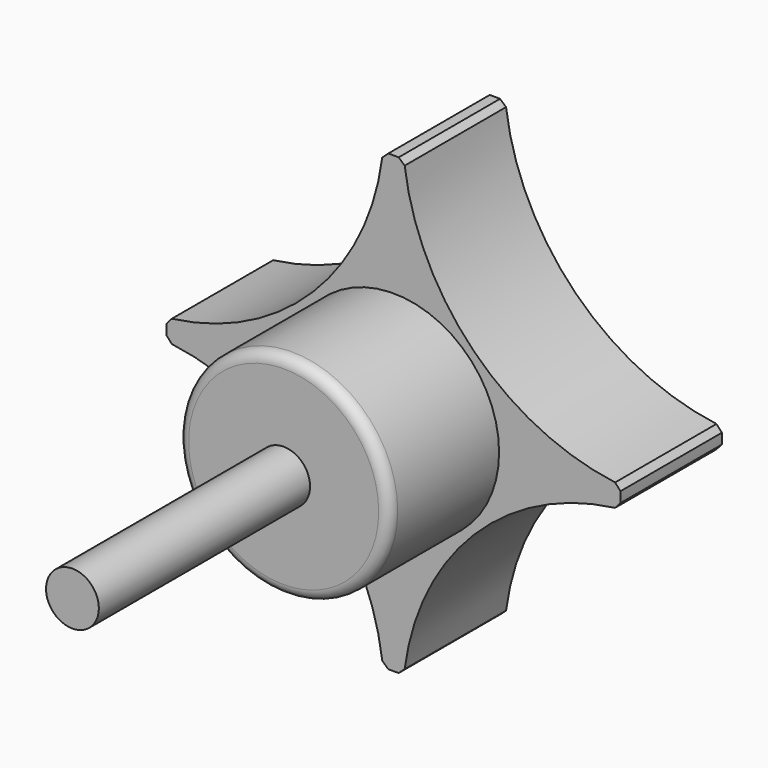
from build123d import *

# Parameters (mm, degrees)
F0_R        = 21.5
F1_DEPTH    = 12
F3_DEPTH    = 12
F4_R        = 10
F5_DEPTH    = 13
F6_R        = 2.5
F7_DEPTH    = 25
F8_T1_DEPTH = 14.6145321273
F9_R        = 1


# Not quite as in the source:
# - a fillet or chamfer that OpenCascade refuses, or shapes differently, is made with other operations: its cross-section is extruded or revolved along the edge and cut away or added


with BuildPart() as f1:
    # F0 (on Front) → F1 (new body)
    with BuildSketch(Plane.XZ):
        Circle(F0_R)
    extrude(amount=F1_DEPTH)

    # F2 (on face) → F3 (cut)
    with BuildSketch(Plane.XZ.offset(12)):
        with BuildLine():
            ThreePointArc((-1, 21.4767315949), (-15.2027957955, 15.2027957955), (-21.4767315949, 1))
            ThreePointArc((-21.4767315949, 1), (-7.6309801067, 7.6309801067), (-1, 21.4767315949))
        make_face()
        with BuildLine():
            ThreePointArc((1, 21.4767315949), (7.6309801067, 7.6309801067), (21.4767315949, 1))
            ThreePointArc((21.4767315949, 1), (15.2027957955, 15.2027957955), (1, 21.4767315949))
        make_face()
        with BuildLine():
            ThreePointArc((-1, -21.4767315949), (-7.6309801067, -7.6309801067), (-21.4767315949, -1))
            ThreePointArc((-21.4767315949, -1), (-15.2027957955, -15.2027957955), (-1, -21.4767315949))
        make_face()
        with BuildLine():
            ThreePointArc((1, -21.4767315949), (15.2027957955, -15.2027957955), (21.4767315949, -1))
            ThreePointArc((21.4767315949, -1), (7.6309801067, -7.6309801067), (1, -21.4767315949))
        make_face()
    extrude(amount=-F3_DEPTH, mode=Mode.SUBTRACT)

    # F4 (on face) → F5 (join)
    with BuildSketch(Plane.XZ.offset(12)):
        Circle(F4_R)
    extrude(amount=F5_DEPTH)

    # F6 (on face) → F7 (join)
    with BuildSketch(Plane.XZ.offset(25)):
        Circle(F6_R)
    extrude(amount=F7_DEPTH)

    # F8: chamfer of 0.5 on 8 edges, made by hand

    # F8_s2 → F8_t1 (cut)
    with BuildSketch(Plane.XZ.offset(-1.3072660637)):
        with BuildLine():
            Line((-0.4780125983, 21.5077200164), (-1.0733486412, 20.9725576393))
            Line((-1.0733486412, 20.9725576393), (-1.0832651887, 20.973846858))
            ThreePointArc((-1.0832651887, 20.973846858), (-1.0387448634, 21.2248919874), (-1.0099418634, 21.4778083267))
            Line((-1.0099418634, 21.4778083267), (-1.0004651163, 21.4867207724))
            ThreePointArc((-1.0004651163, 21.4867207724), (-0.7391806182, 21.4972954581), (-0.4782418478, 21.5177173883))
            Line((-0.4782418478, 21.5177173883), (-0.4780125983, 21.5077200164))
        make_face()
        with BuildLine():
            Line((-20.9725576393, 1.0733486412), (-21.5077200164, 0.4780125983))
            Line((-21.5077200164, 0.4780125983), (-21.5177173883, 0.4782418478))
            ThreePointArc((-21.5177173883, 0.4782418478), (-21.4972954581, 0.7391806182), (-21.4867207724, 1.0004651163))
            Line((-21.4867207724, 1.0004651163), (-21.4778083267, 1.0099418634))
            ThreePointArc((-21.4778083267, 1.0099418634), (-21.2248919874, 1.0387448634), (-20.973846858, 1.0832651887))
            Line((-20.973846858, 1.0832651887), (-20.9725576393, 1.0733486412))
        make_face()
        with BuildLine():
            Line((-21.5077200164, -0.4780125983), (-20.9725576393, -1.0733486412))
            Line((-20.9725576393, -1.0733486412), (-20.973846858, -1.0832651887))
            ThreePointArc((-20.973846858, -1.0832651887), (-21.2248919874, -1.0387448634), (-21.4778083267, -1.0099418634))
            Line((-21.4778083267, -1.0099418634), (-21.4867207724, -1.0004651163))
            ThreePointArc((-21.4867207724, -1.0004651163), (-21.4972954581, -0.7391806182), (-21.5177173883, -0.4782418478))
            Line((-21.5177173883, -0.4782418478), (-21.5077200164, -0.4780125983))
        make_face()
        with BuildLine():
            Line((1.0733486412, 20.9725576393), (0.4780125983, 21.5077200164))
            Line((0.4780125983, 21.5077200164), (0.4782418478, 21.5177173883))
            ThreePointArc((0.4782418478, 21.5177173883), (0.7391806182, 21.4972954581), (1.0004651163, 21.4867207724))
            Line((1.0004651163, 21.4867207724), (1.0099418634, 21.4778083267))
            ThreePointArc((1.0099418634, 21.4778083267), (1.0387448634, 21.2248919874), (1.0832651887, 20.973846858))
            Line((1.0832651887, 20.973846858), (1.0733486412, 20.9725576393))
        make_face()
        with BuildLine():
            Line((21.5077200164, 0.4780125983), (20.9725576393, 1.0733486412))
            Line((20.9725576393, 1.0733486412), (20.973846858, 1.0832651887))
            ThreePointArc((20.973846858, 1.0832651887), (21.2248919874, 1.0387448634), (21.4778083267, 1.0099418634))
            Line((21.4778083267, 1.0099418634), (21.4867207724, 1.0004651163))
            ThreePointArc((21.4867207724, 1.0004651163), (21.4972954581, 0.7391806182), (21.5177173883, 0.4782418478))
            Line((21.5177173883, 0.4782418478), (21.5077200164, 0.4780125983))
        make_face()
        with BuildLine():
            Line((1.0733486412, -20.9725576393), (0.4780125983, -21.5077200164))
            Line((0.4780125983, -21.5077200164), (0.4782418478, -21.5177173883))
            ThreePointArc((0.4782418478, -21.5177173883), (0.7391806182, -21.4972954581), (1.0004651163, -21.4867207724))
            Line((1.0004651163, -21.4867207724), (1.0099418634, -21.4778083267))
            ThreePointArc((1.0099418634, -21.4778083267), (1.0387448634, -21.2248919874), (1.0832651887, -20.973846858))
            Line((1.0832651887, -20.973846858), (1.0733486412, -20.9725576393))
        make_face()
        with BuildLine():
            Line((-1.0733486412, -20.9725576393), (-0.4780125983, -21.5077200164))
            Line((-0.4780125983, -21.5077200164), (-0.4782418478, -21.5177173883))
            ThreePointArc((-0.4782418478, -21.5177173883), (-0.7391806182, -21.4972954581), (-1.0004651163, -21.4867207724))
            Line((-1.0004651163, -21.4867207724), (-1.0099418634, -21.4778083267))
            ThreePointArc((-1.0099418634, -21.4778083267), (-1.0387448634, -21.2248919874), (-1.0832651887, -20.973846858))
            Line((-1.0832651887, -20.973846858), (-1.0733486412, -20.9725576393))
        make_face()
        with BuildLine():
            Line((21.5077200164, -0.4780125983), (20.9725576393, -1.0733486412))
            Line((20.9725576393, -1.0733486412), (20.973846858, -1.0832651887))
            ThreePointArc((20.973846858, -1.0832651887), (21.2248919874, -1.0387448634), (21.4778083267, -1.0099418634))
            Line((21.4778083267, -1.0099418634), (21.4867207724, -1.0004651163))
            ThreePointArc((21.4867207724, -1.0004651163), (21.4972954581, -0.7391806182), (21.5177173883, -0.4782418478))
            Line((21.5177173883, -0.4782418478), (21.5077200164, -0.4780125983))
        make_face()
    extrude(amount=F8_T1_DEPTH, mode=Mode.SUBTRACT)

    # F9
    f9_edges = [f1.edges().sort_by_distance(p)[0] for p in [
        (-10, -25, 0),
    ]]
    fillet(f9_edges, radius=F9_R)


solid = f1.part
